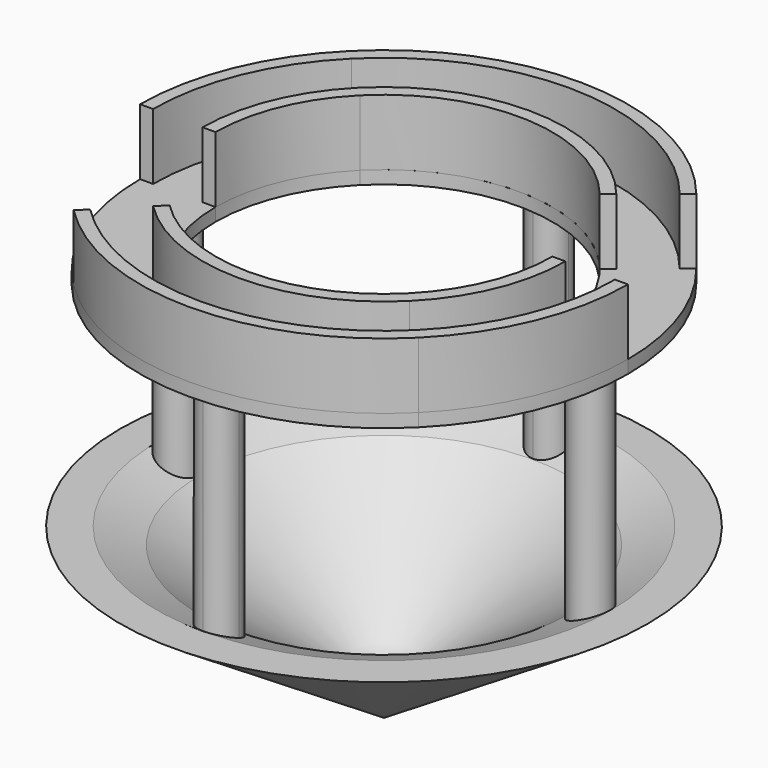
from build123d import *

# Parameters (mm, degrees)
F1_DEPTH = 12.7
F2_DEPTH = 2.5
F4_DEPTH = 44.45


# Not quite as in the source:
# - a length typed as a fraction of an inch, garbled in the dataset ("3 / 203.2 mm" for 3/8 in), is restored


with BuildPart() as f1:
    # F0 (on Top) → F1 (new body)
    with BuildSketch(Plane.XY):
        with BuildLine():
            Line((33.1977999888, -33.1995267422), (31.4300790096, -31.4317138166))
            ThreePointArc((31.4300790096, -31.4317138166), (0, -44.45), (-31.4300790096, -31.4317138166))
            Line((-31.4300790096, -31.4317138166), (-33.1977999888, -33.1995267422))
            ThreePointArc((-33.1977999888, -33.1995267422), (0, -46.95), (33.1977999888, -33.1995267422))
        make_face()
        with BuildLine():
            Line((46.95, 0), (44.45, 0))
            ThreePointArc((44.45, 0), (41.0662240289, -17.0108125618), (31.4300790096, -31.4317138166))
            Line((31.4300790096, -31.4317138166), (33.1977999888, -33.1995267422))
            ThreePointArc((33.1977999888, -33.1995267422), (43.3759104197, -17.967551176), (46.95, 0))
        make_face()
    extrude(amount=F1_DEPTH)


with BuildPart() as f1b:
    # F0 (on Top) → F1, piece 2 (new body)
    with BuildSketch(Plane.XY):
        with BuildLine():
            ThreePointArc((-31.4300790096, 31.4317138166), (2.3760514819, 44.3864492763), (34.6059908934, 27.8967362658))
            Line((34.6059908934, 27.8967362658), (36.5523345882, 29.4657315563))
            ThreePointArc((36.5523345882, 29.4657315563), (2.5096876732, 46.8828749949), (-33.1977999888, 33.1995267422))
            Line((-33.1977999888, 33.1995267422), (-31.4300790096, 31.4317138166))
        make_face()
        with BuildLine():
            ThreePointArc((-44.45, 0), (-41.0662240289, 17.0108125618), (-31.4300790096, 31.4317138166))
            Line((-31.4300790096, 31.4317138166), (-33.1977999888, 33.1995267422))
            ThreePointArc((-33.1977999888, 33.1995267422), (-43.3759104197, 17.967551176), (-46.95, 0))
            Line((-46.95, 0), (-44.45, 0))
        make_face()
    extrude(amount=F1_DEPTH)


with BuildPart() as f1c:
    # F0 (on Top) → F1, piece 3 (new body)
    with BuildSketch(Plane.XY):
        with BuildLine():
            ThreePointArc((-24.695062079, -24.6963465702), (0, -34.925), (24.695062079, -24.6963465702))
            Line((24.695062079, -24.6963465702), (23.4743895005, -23.4756104995))
            Line((23.4743895005, -23.4756104995), (22.9273410998, -22.9285336446))
            ThreePointArc((22.9273410998, -22.9285336446), (0, -32.425), (-22.9273410998, -22.9285336446))
            Line((-22.9273410998, -22.9285336446), (-24.695062079, -24.6963465702))
        make_face()
        with BuildLine():
            ThreePointArc((24.695062079, -24.6963465702), (32.2663188798, -13.3656384414), (34.925, 0))
            Line((34.925, 0), (32.425, 0))
            ThreePointArc((32.425, 0), (29.956632489, -12.4088998271), (22.9273410998, -22.9285336446))
            Line((22.9273410998, -22.9285336446), (23.4743895005, -23.4756104995))
            Line((23.4743895005, -23.4756104995), (24.695062079, -24.6963465702))
        make_face()
    extrude(amount=F1_DEPTH)


with BuildPart() as f1d:
    # F0 (on Top) → F1, piece 4 (new body)
    with BuildSketch(Plane.XY):
        with BuildLine():
            Line((25.2440777215, 20.3498689183), (27.1904214163, 21.9188642088))
            ThreePointArc((27.1904214163, 21.9188642088), (1.8668975929, 34.8750672885), (-24.695062079, 24.6963465702))
            Line((-24.695062079, 24.6963465702), (-22.9273410998, 22.9285336446))
            ThreePointArc((-22.9273410998, 22.9285336446), (1.7332614016, 32.3786415699), (25.2440777215, 20.3498689183))
        make_face()
        with BuildLine():
            Line((-22.9273410998, 22.9285336446), (-24.695062079, 24.6963465702))
            ThreePointArc((-24.695062079, 24.6963465702), (-32.2663188798, 13.3656384414), (-34.925, 0))
            Line((-34.925, 0), (-32.425, 0))
            ThreePointArc((-32.425, 0), (-29.956632489, 12.4088998271), (-22.9273410998, 22.9285336446))
        make_face()
    extrude(amount=F1_DEPTH)


with BuildPart() as f2:
    # F0 (on Top) → F2 (new body)
    with BuildSketch(Plane.XY):
        with BuildLine():
            Line((-33.1977999888, -33.1995267422), (-31.4300790096, -31.4317138166))
            ThreePointArc((-31.4300790096, -31.4317138166), (-41.0662240289, -17.0108125618), (-44.45, 0))
            Line((-44.45, 0), (-46.95, 0))
            ThreePointArc((-46.95, 0), (-43.3759104197, -17.967551176), (-33.1977999888, -33.1995267422))
        make_face()
        with BuildLine():
            Line((33.1977999888, -33.1995267422), (31.4300790096, -31.4317138166))
            ThreePointArc((31.4300790096, -31.4317138166), (0, -44.45), (-31.4300790096, -31.4317138166))
            Line((-31.4300790096, -31.4317138166), (-33.1977999888, -33.1995267422))
            ThreePointArc((-33.1977999888, -33.1995267422), (0, -46.95), (33.1977999888, -33.1995267422))
        make_face()
        with BuildLine():
            Line((-31.4300790096, -31.4317138166), (-24.695062079, -24.6963465702))
            ThreePointArc((-24.695062079, -24.6963465702), (-32.2663188798, -13.3656384414), (-34.925, 0))
            Line((-34.925, 0), (-44.45, 0))
            ThreePointArc((-44.45, 0), (-41.0662240289, -17.0108125618), (-31.4300790096, -31.4317138166))
        make_face()
        with BuildLine():
            Line((31.4300790096, -31.4317138166), (24.695062079, -24.6963465702))
            ThreePointArc((24.695062079, -24.6963465702), (0, -34.925), (-24.695062079, -24.6963465702))
            Line((-24.695062079, -24.6963465702), (-31.4300790096, -31.4317138166))
            ThreePointArc((-31.4300790096, -31.4317138166), (0, -44.45), (31.4300790096, -31.4317138166))
        make_face()
        with BuildLine():
            Line((44.45, 0), (34.925, 0))
            ThreePointArc((34.925, 0), (32.2663188798, -13.3656384414), (24.695062079, -24.6963465702))
            Line((24.695062079, -24.6963465702), (31.4300790096, -31.4317138166))
            ThreePointArc((31.4300790096, -31.4317138166), (41.0662240289, -17.0108125618), (44.45, 0))
        make_face()
        with BuildLine():
            ThreePointArc((-24.695062079, -24.6963465702), (0, -34.925), (24.695062079, -24.6963465702))
            Line((24.695062079, -24.6963465702), (23.4743895005, -23.4756104995))
            Line((23.4743895005, -23.4756104995), (22.9273410998, -22.9285336446))
            ThreePointArc((22.9273410998, -22.9285336446), (0, -32.425), (-22.9273410998, -22.9285336446))
            Line((-22.9273410998, -22.9285336446), (-24.695062079, -24.6963465702))
        make_face()
        with BuildLine():
            ThreePointArc((-34.925, 0), (-32.2663188798, -13.3656384414), (-24.695062079, -24.6963465702))
            Line((-24.695062079, -24.6963465702), (-22.9273410998, -22.9285336446))
            ThreePointArc((-22.9273410998, -22.9285336446), (-29.956632489, -12.4088998271), (-32.425, 0))
            Line((-32.425, 0), (-34.925, 0))
        make_face()
        with BuildLine():
            ThreePointArc((24.695062079, -24.6963465702), (32.2663188798, -13.3656384414), (34.925, 0))
            Line((34.925, 0), (32.425, 0))
            ThreePointArc((32.425, 0), (29.956632489, -12.4088998271), (22.9273410998, -22.9285336446))
            Line((22.9273410998, -22.9285336446), (23.4743895005, -23.4756104995))
            Line((23.4743895005, -23.4756104995), (24.695062079, -24.6963465702))
        make_face()
        with BuildLine():
            Line((46.95, 0), (44.45, 0))
            ThreePointArc((44.45, 0), (41.0662240289, -17.0108125618), (31.4300790096, -31.4317138166))
            Line((31.4300790096, -31.4317138166), (33.1977999888, -33.1995267422))
            ThreePointArc((33.1977999888, -33.1995267422), (43.3759104197, -17.967551176), (46.95, 0))
        make_face()
        with BuildLine():
            ThreePointArc((34.6059908934, 27.8967362658), (41.9168152131, 14.7913184806), (44.45, 0))
            Line((44.45, 0), (46.95, 0))
            ThreePointArc((46.95, 0), (44.274341378, 15.6232261566), (36.5523345882, 29.4657315563))
            Line((36.5523345882, 29.4657315563), (34.6059908934, 27.8967362658))
        make_face()
        with BuildLine():
            ThreePointArc((27.1904214163, 21.9188642088), (32.9346405246, 11.6217502347), (34.925, 0))
            Line((34.925, 0), (44.45, 0))
            ThreePointArc((44.45, 0), (41.9168152131, 14.7913184806), (34.6059908934, 27.8967362658))
            Line((34.6059908934, 27.8967362658), (27.1904214163, 21.9188642088))
        make_face()
        with BuildLine():
            Line((32.425, 0), (34.925, 0))
            ThreePointArc((34.925, 0), (32.9346405246, 11.6217502347), (27.1904214163, 21.9188642088))
            Line((27.1904214163, 21.9188642088), (25.2440777215, 20.3498689183))
            ThreePointArc((25.2440777215, 20.3498689183), (30.5771143596, 10.7898425587), (32.425, 0))
        make_face()
        with BuildLine():
            ThreePointArc((-24.695062079, 24.6963465702), (1.8668975929, 34.8750672885), (27.1904214163, 21.9188642088))
            Line((27.1904214163, 21.9188642088), (34.6059908934, 27.8967362658))
            ThreePointArc((34.6059908934, 27.8967362658), (2.3760514819, 44.3864492763), (-31.4300790096, 31.4317138166))
            Line((-31.4300790096, 31.4317138166), (-24.695062079, 24.6963465702))
        make_face()
        with BuildLine():
            ThreePointArc((-34.925, 0), (-32.2663188798, 13.3656384414), (-24.695062079, 24.6963465702))
            Line((-24.695062079, 24.6963465702), (-31.4300790096, 31.4317138166))
            ThreePointArc((-31.4300790096, 31.4317138166), (-41.0662240289, 17.0108125618), (-44.45, 0))
            Line((-44.45, 0), (-34.925, 0))
        make_face()
        with BuildLine():
            Line((-22.9273410998, 22.9285336446), (-24.695062079, 24.6963465702))
            ThreePointArc((-24.695062079, 24.6963465702), (-32.2663188798, 13.3656384414), (-34.925, 0))
            Line((-34.925, 0), (-32.425, 0))
            ThreePointArc((-32.425, 0), (-29.956632489, 12.4088998271), (-22.9273410998, 22.9285336446))
        make_face()
        with BuildLine():
            Line((25.2440777215, 20.3498689183), (27.1904214163, 21.9188642088))
            ThreePointArc((27.1904214163, 21.9188642088), (1.8668975929, 34.8750672885), (-24.695062079, 24.6963465702))
            Line((-24.695062079, 24.6963465702), (-22.9273410998, 22.9285336446))
            ThreePointArc((-22.9273410998, 22.9285336446), (1.7332614016, 32.3786415699), (25.2440777215, 20.3498689183))
        make_face()
        with BuildLine():
            ThreePointArc((-44.45, 0), (-41.0662240289, 17.0108125618), (-31.4300790096, 31.4317138166))
            Line((-31.4300790096, 31.4317138166), (-33.1977999888, 33.1995267422))
            ThreePointArc((-33.1977999888, 33.1995267422), (-43.3759104197, 17.967551176), (-46.95, 0))
            Line((-46.95, 0), (-44.45, 0))
        make_face()
        with BuildLine():
            ThreePointArc((-31.4300790096, 31.4317138166), (2.3760514819, 44.3864492763), (34.6059908934, 27.8967362658))
            Line((34.6059908934, 27.8967362658), (36.5523345882, 29.4657315563))
            ThreePointArc((36.5523345882, 29.4657315563), (2.5096876732, 46.8828749949), (-33.1977999888, 33.1995267422))
            Line((-33.1977999888, 33.1995267422), (-31.4300790096, 31.4317138166))
        make_face()
    extrude(amount=-F2_DEPTH)

    # F3 (on face) → F4 (join)
    with BuildSketch(Plane(origin=(0, 0, -2.5), x_dir=(1, 0, 0), z_dir=(0, 0, -1))):
        with BuildLine():
            Line((0, 39.6875), (0, 43.4975))
            ThreePointArc((0, 43.4975), (-3.81, 39.6875), (0, 35.8775))
            Line((0, 35.8775), (0, 39.6875))
        make_face()
        with BuildLine():
            ThreePointArc((3.81, 39.6875), (2.6940768363, 42.3815768363), (0, 43.4975))
            Line((0, 43.4975), (0, 39.6875))
            Line((0, 39.6875), (0, 35.8775))
            ThreePointArc((0, 35.8775), (2.6940768363, 36.9934231637), (3.81, 39.6875))
        make_face()
        with BuildLine():
            Line((35.8775, 0), (43.4975, 0))
            ThreePointArc((43.4975, 0), (39.6875, 3.81), (35.8775, 0))
        make_face()
        with BuildLine():
            ThreePointArc((35.8775, 0), (39.6875, -3.81), (43.4975, 0))
            Line((43.4975, 0), (35.8775, 0))
        make_face()
        with BuildLine():
            ThreePointArc((-35.8775, 0), (-39.6875, 3.81), (-43.4975, 0))
            Line((-43.4975, 0), (-35.8775, 0))
        make_face()
        with BuildLine():
            Line((-35.8775, 0), (-43.4975, 0))
            ThreePointArc((-43.4975, 0), (-39.6875, -3.81), (-35.8775, 0))
        make_face()
        with BuildLine():
            ThreePointArc((0, -35.8775), (-3.81, -39.6875), (0, -43.4975))
            Line((0, -43.4975), (0, -35.8775))
        make_face()
        with BuildLine():
            Line((0, -35.8775), (0, -43.4975))
            ThreePointArc((0, -43.4975), (2.6940768363, -42.3815768363), (3.81, -39.6875))
            ThreePointArc((3.81, -39.6875), (2.6940768363, -36.9934231637), (0, -35.8775))
        make_face()
    extrude(amount=F4_DEPTH)

    # F5 (on Front) → F6 (revolve)
    with BuildSketch(Plane.XZ):
        Polygon((0, -76.0341584682), (50.8, -43.5579530895), (43.7318012118, -43.5579530895), (35.7412993908, -46.7542223632), (0, -72.013489902), align=None)
    revolve(axis=Axis((0, 0, -74.0238241851), (0, 0, 1)))


solid = Compound([f1.part, f1b.part, f1c.part, f1d.part, f2.part])
